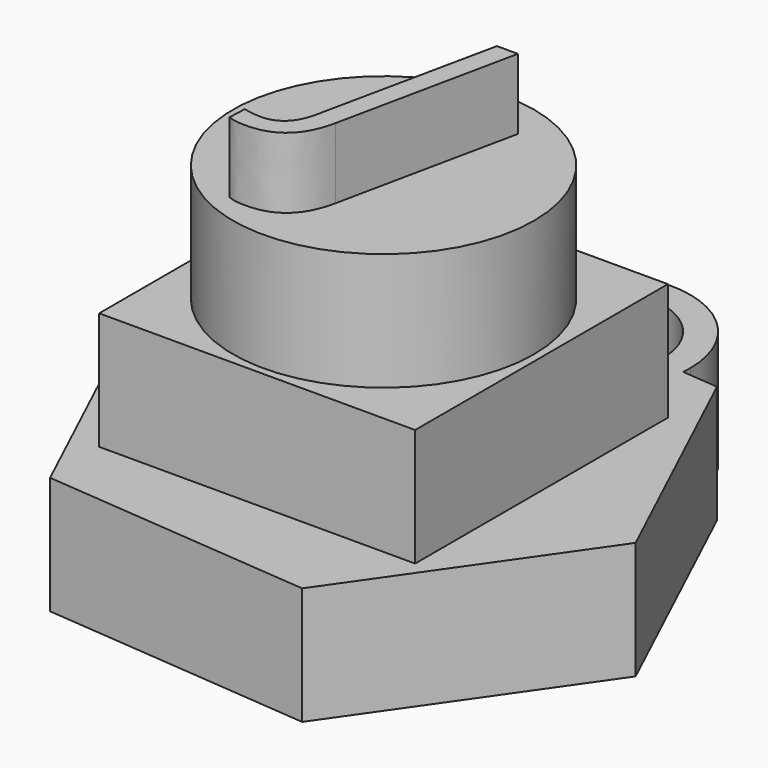
from build123d import *

# Parameters (mm, degrees)
F1_DEPTH      = 6.35
F2_W          = 17.0635422
F2_H          = 17.0635422
F4_DEPTH      = 6.35
F3_R          = 8.1294361085
F5_DEPTH      = 12.7
F6_TEXT_SIZE  = 13.611805884
F7_DEPTH      = 3.81
F9_DEPTH      = 6.35
F10_TEXT_SIZE = 16.8955357165
F11_DEPTH     = 5.08
F12_TEXT_SIZE = 14.7819965302
F13_DEPTH     = 6.35


# Not quite as in the source:
# - Text() gives the source's letters only with a copy of the font that has no kerning and outlines rounded to 1/6400 em; it was checked with that copy


with BuildPart() as f1:
    # F0 (on Top) → F1 (new body)
    with BuildSketch(Plane.XY):
        Polygon((6.2264752225, -13.2772112899), (14.6116398797, -1.2463199262), (8.3851646572, 12.0308913637), (-6.2264752225, 13.2772112899), (-14.6116398797, 1.2463199262), (-8.3851646572, -12.0308913637), align=None)
    extrude(amount=F1_DEPTH)

    # F2 (on face) → F4 (join)
    with BuildSketch(Plane.XY.offset(6.35)):
        Rectangle(F2_W, F2_H)
    extrude(amount=F4_DEPTH)

    # F3 (on face) → F5 (join)
    with BuildSketch(Plane.XY.offset(6.35)):
        Circle(F3_R)
    extrude(amount=F5_DEPTH)

    # F6 (on face) → F7 (join)
    with BuildSketch(Plane.XY.offset(19.05)):
        with Locations((-1.1121122094, -3.9524988043)):
            Text('J', F6_TEXT_SIZE, font='Open Sans', font_style=FontStyle.ITALIC, text_align=(TextAlign.LEFT, TextAlign.BOTTOM))
    extrude(amount=F7_DEPTH)

    # F8 (on face) → F9 (join)
    with BuildSketch(Plane(origin=(0, 0, 0), x_dir=(1, 0, 0), z_dir=(0, 0, -1))):
        with BuildLine():
            ThreePointArc((-4.2652974004, -13.1099299294), (1.3074904702, -18.0132466192), (6.4433939963, -12.6540513268))
            ThreePointArc((6.4433939963, -12.6540513268), (6.4385400098, -12.4259055739), (6.4239868351, -12.1981727242))
            Line((6.4239868351, -12.1981727242), (4.9521099735, -12.3237184861))
            ThreePointArc((4.9521099735, -12.3237184861), (4.9626553062, -12.4887353102), (4.9661725389, -12.6540513268))
            ThreePointArc((4.9661725389, -12.6540513268), (1.2446607339, -16.5373619156), (-2.7934205388, -12.9843841675))
            Line((-2.7934205388, -12.9843841675), (-4.2652974004, -13.1099299294))
        make_face()
    extrude(amount=-F9_DEPTH)

    # F10 (on face) → F11 (join)
    with BuildSketch(Plane(origin=(0, 0, 0), x_dir=(1, 0, 0), z_dir=(0, 0, -1))):
        with Locations((-6.3285953365, -6.7724999972)):
            Text('X', F10_TEXT_SIZE, font='Open Sans', text_align=(TextAlign.LEFT, TextAlign.BOTTOM))
    extrude(amount=-F11_DEPTH)

    # F12 (on face) → F13 (cut)
    with BuildSketch(Plane(origin=(0, 0, 0), x_dir=(1, 0, 0), z_dir=(0, 0, -1))):
        with Locations((-6.2264752225, -5.5024451576)):
            Text('X', F12_TEXT_SIZE, font='Open Sans', text_align=(TextAlign.LEFT, TextAlign.BOTTOM))
    extrude(amount=-F13_DEPTH, mode=Mode.SUBTRACT)


solid = f1.part
